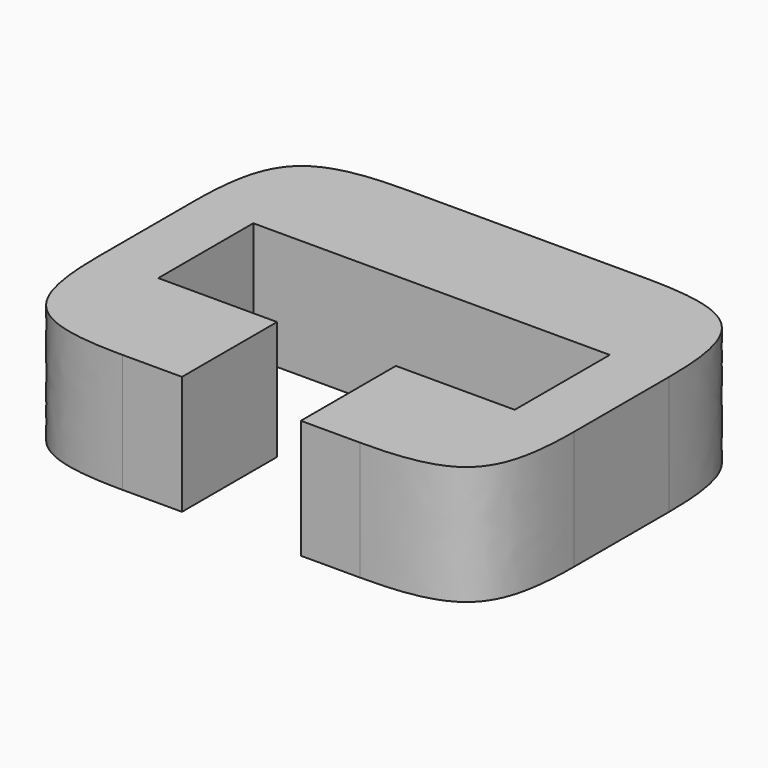
from build123d import *

# Parameters (mm, degrees)
F2_DEPTH    = 6.35
F3_T1_DEPTH = 76.2


# Not quite as in the source:
# - a variable given as a bare number and used for a length is read in inches; the dataset says mm whatever the document's units were
# - a fillet or chamfer that OpenCascade refuses, or shapes differently, is made with other operations: its cross-section is extruded or revolved along the edge and cut away or added


with BuildPart() as f2:
    # F1 (on Top) → F2 (new body, symmetric)
    with BuildSketch(Plane.XY):
        Polygon((25.4, 19.05), (-25.4, 19.05), (-25.4, -19.05), (-6.35, -19.05), (-6.35, -6.35), (-19.05, -6.35), (-19.05, 6.35), (19.05, 6.35), (19.05, -6.35), (6.35, -6.35), (6.35, -19.05), (25.4, -19.05), align=None)
    extrude(amount=F2_DEPTH, both=True)

    # F3: fillet of radius 12.7 on 4 edges, made by hand

    # F3_s2 → F3_t1 (cut)
    with BuildSketch(Plane.XY.offset(-38.1)):
        with BuildLine():
            add(Edge.make_bspline(
                [(25.4, -6.35), (25.4, -19.05), (12.7, -19.05)],
                knots=[0, 0, 0, 1, 1, 1], degree=2, weights=[1, 1.5, 1]))
            Line((12.7, -19.05), (25.4, -19.05))
            Line((25.4, -19.05), (25.4, -6.35))
        make_face()
        with BuildLine():
            add(Edge.make_bspline(
                [(12.7, 19.05), (25.4, 19.05), (25.4, 6.35)],
                knots=[0, 0, 0, 1, 1, 1], degree=2, weights=[1, 1.5, 1]))
            Line((25.4, 6.35), (25.4, 19.05))
            Line((25.4, 19.05), (12.7, 19.05))
        make_face()
        with BuildLine():
            add(Edge.make_bspline(
                [(-25.4, 6.35), (-25.4, 19.05), (-12.7, 19.05)],
                knots=[0, 0, 0, 1, 1, 1], degree=2, weights=[1, 1.5, 1]))
            Line((-12.7, 19.05), (-25.4, 19.05))
            Line((-25.4, 19.05), (-25.4, 6.35))
        make_face()
        with BuildLine():
            add(Edge.make_bspline(
                [(-12.7, -19.05), (-25.4, -19.05), (-25.4, -6.35)],
                knots=[0, 0, 0, 1, 1, 1], degree=2, weights=[1, 1.5, 1]))
            Line((-25.4, -6.35), (-25.4, -19.05))
            Line((-25.4, -19.05), (-12.7, -19.05))
        make_face()
    extrude(amount=F3_T1_DEPTH, mode=Mode.SUBTRACT)


solid = f2.part
